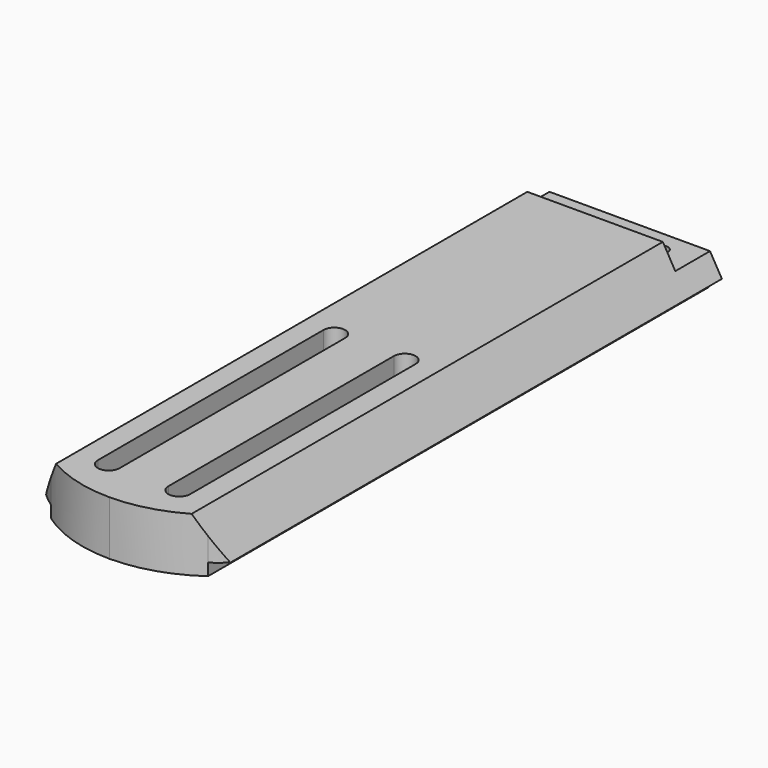
from build123d import *

# Parameters (mm, degrees)
F1_DEPTH = 60
F3_DEPTH = 25
F5_DEPTH = 5.5
F7_DEPTH = 25
F9_DEPTH = 4
F11_D    = 2.5


with BuildPart() as f1:
    # F0 (on Front) → F1 (new body, symmetric)
    with BuildSketch(Plane.XZ):
        Polygon((-14.5, 2.2), (-14.5, 0), (14.5, 0), (14.5, 2.2), (17.0033320997, 2.2), (12.5, 10), (-12.5, 10), (-17.0033320997, 2.2), align=None)
    extrude(amount=F1_DEPTH, both=True)

    # F2 (on face) → F3 (cut)
    with BuildSketch(Plane.XY.offset(10)):
        with BuildLine():
            ThreePointArc((-4.5, 0), (-6.5, 2), (-8.5, 0))
            Line((-8.5, 0), (-8.5, -52))
            ThreePointArc((-8.5, -52), (-6.5, -54), (-4.5, -52))
            Line((-4.5, -52), (-4.5, 0))
        make_face()
        with BuildLine():
            ThreePointArc((8.5, 0), (6.5, 2), (4.5, 0))
            Line((4.5, 0), (4.5, -52))
            ThreePointArc((4.5, -52), (6.5, -54), (8.5, -52))
            Line((8.5, -52), (8.5, 0))
        make_face()
    extrude(amount=-F3_DEPTH, mode=Mode.SUBTRACT)

    # F4 (on face) → F5 (cut)
    with BuildSketch(Plane(origin=(0, 0, 0), x_dir=(1, 0, 0), z_dir=(0, 0, -1))):
        with BuildLine():
            ThreePointArc((-10.5, 0), (-6.5, -4), (-2.5, 0))
            Line((-2.5, 0), (-2.5, 52))
            ThreePointArc((-2.5, 52), (-6.5, 56), (-10.5, 52))
            Line((-10.5, 52), (-10.5, 0))
        make_face()
        with BuildLine():
            ThreePointArc((-4.5, 0), (-6.5, -2), (-8.5, 0))
            Line((-8.5, 0), (-8.5, 52))
            ThreePointArc((-8.5, 52), (-6.5, 54), (-4.5, 52))
            Line((-4.5, 52), (-4.5, 0))
        make_face(mode=Mode.SUBTRACT)
        with BuildLine():
            ThreePointArc((2.5, 0), (6.5, -4), (10.5, 0))
            Line((10.5, 0), (10.5, 52))
            ThreePointArc((10.5, 52), (6.5, 56), (2.5, 52))
            Line((2.5, 52), (2.5, 0))
        make_face()
        with BuildLine():
            ThreePointArc((4.5, 52), (6.5, 54), (8.5, 52))
            Line((8.5, 52), (8.5, 0))
            ThreePointArc((8.5, 0), (6.5, -2), (4.5, 0))
            Line((4.5, 0), (4.5, 52))
        make_face(mode=Mode.SUBTRACT)
    extrude(amount=-F5_DEPTH, mode=Mode.SUBTRACT)

    # F6 (on face) → F7 (cut)
    with BuildSketch(Plane(origin=(0, 0, 0), x_dir=(1, 0, 0), z_dir=(0, 0, -1))):
        with BuildLine():
            ThreePointArc((0, 60), (7.6113304895, 58.8131822355), (14.5, 55.3654118544))
            Line((14.5, 55.3654118544), (14.5, 60))
            Line((14.5, 60), (0, 60))
        make_face()
        with BuildLine():
            ThreePointArc((-14.5, 55.3654118544), (-7.6113304895, 58.8131822355), (0, 60))
            Line((0, 60), (-14.5, 60))
            Line((-14.5, 60), (-14.5, 55.3654118544))
        make_face()
        with BuildLine():
            ThreePointArc((14.5, 55.3654118544), (18.1961519016, 52.1435135248), (21.1923439056, 48.2621476311))
            Line((21.1923439056, 48.2621476311), (21.1923439056, 66.2593638897))
            Line((21.1923439056, 66.2593638897), (-20.7064654678, 66.2593638897))
            Line((-20.7064654678, 66.2593638897), (-20.7064654678, 49.0086504643))
            ThreePointArc((-20.7064654678, 49.0086504643), (-17.8878703743, 52.4649389771), (-14.5, 55.3654118544))
            Line((-14.5, 55.3654118544), (-14.5, 60))
            Line((-14.5, 60), (0, 60))
            Line((0, 60), (14.5, 60))
            Line((14.5, 60), (14.5, 55.3654118544))
        make_face()
    extrude(amount=-F7_DEPTH, mode=Mode.SUBTRACT)

    # F8 (on face) → F9 (cut)
    with BuildSketch(Plane.XY.offset(10)):
        Polygon((12.5, 60), (-12.5, 60), (-26.1883419007, 60), (-26.1883419007, 52), (21.1705399538, 52), (21.1705399538, 60), align=None)
    extrude(amount=-F9_DEPTH, mode=Mode.SUBTRACT)

    # F11 (through all)
    with Locations(Plane.XY.offset(6)):
        with Locations((9, 56), (-9, 56)):
            Hole(F11_D / 2)


solid = f1.part
